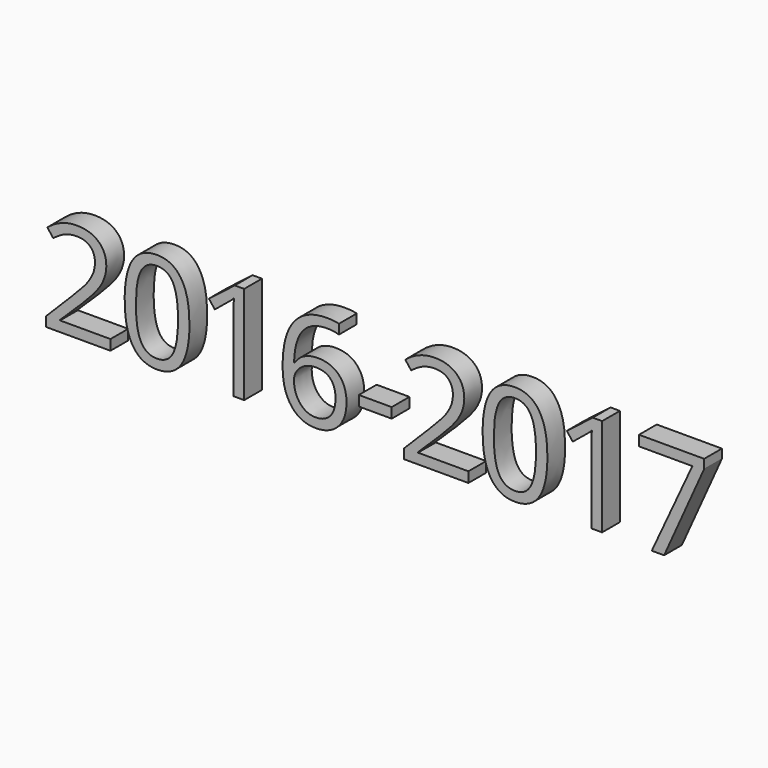
from build123d import *

# Parameters (mm, degrees)
F0_TEXT_SIZE = 39.2468193442
F1_DEPTH     = 6.35


# Not quite as in the source:
# - Text() gives the source's letters only with a copy of the font that has no kerning and outlines rounded to 1/6400 em; it was checked with that copy


with BuildPart() as f1:
    # F0 (on Front) → F1 (new body)
    with BuildSketch(Plane.XZ):
        with Locations((-95.5364219844, -19.0244866535)):
            Text('2016-2017', F0_TEXT_SIZE, font='Open Sans', text_align=(TextAlign.LEFT, TextAlign.BOTTOM))
    extrude(amount=F1_DEPTH)


solid = f1.part
